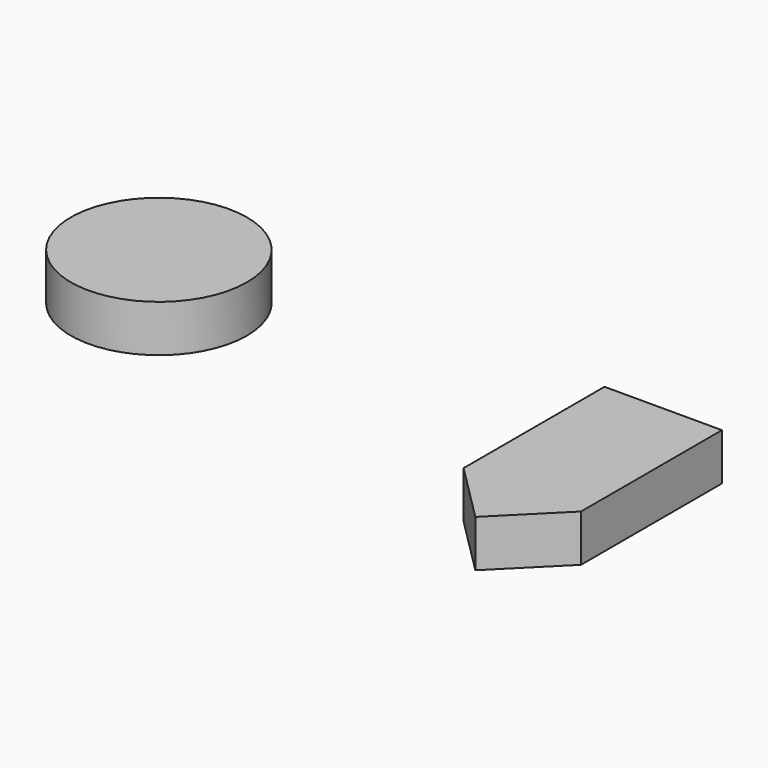
from build123d import *

# Parameters (mm, degrees)
F0_W     = 12.7
F0_H     = 25.4
F1_DEPTH = 5.08
F2_SIZE  = 6.34999
F3_R     = 9.525
F4_DEPTH = 5.08


# Not quite as in the source:
# - a fillet or chamfer is up to 0.001 mm smaller than in the source, because OpenCascade refuses the exact size


with BuildPart() as f1:
    # F0 (on Top) → F1 (new body)
    with BuildSketch(Plane.XY):
        with Locations((0.5088095786, 3.5865946344)):
            Rectangle(F0_W, F0_H)
    extrude(amount=F1_DEPTH)

    # F2 (size 6.35 in the source; OpenCascade refuses exactly that, so slightly less here)
    f2_edges = [f1.edges().sort_by_distance(p)[0] for p in [
        (6.85881, -9.113405, 2.54),
        (-5.84119, -9.113405, 2.54),
    ]]
    chamfer(f2_edges, length=F2_SIZE)


with BuildPart() as f4:
    # F3 (on Top) → F4 (new body)
    with BuildSketch(Plane.XY):
        with Locations((-50.8807636797, 12.3385852203)):
            Circle(F3_R)
    extrude(amount=F4_DEPTH)


solid = Compound([f1.part, f4.part])
